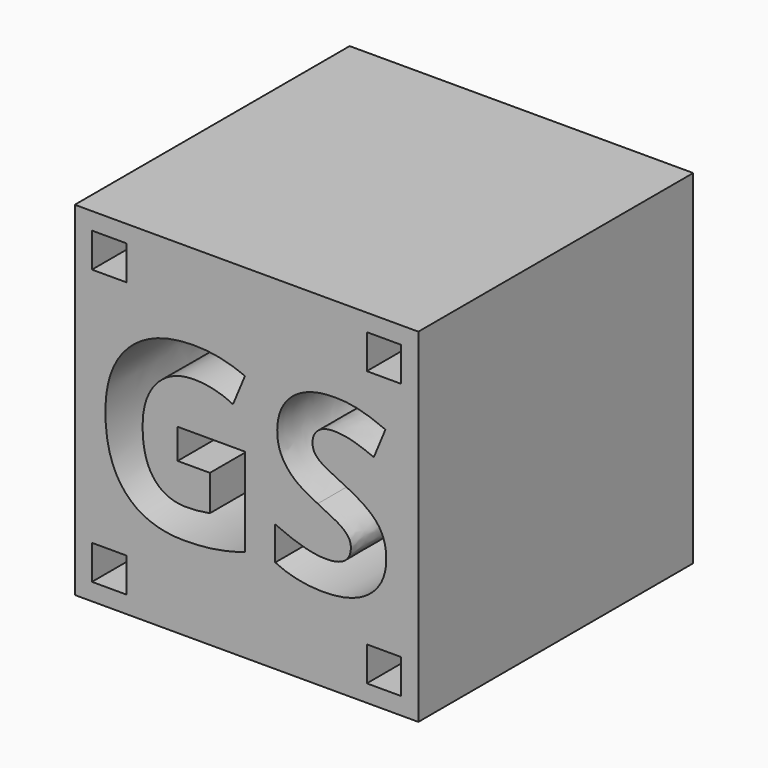
from build123d import *

# Parameters (mm, degrees)
F0_W         = 25.4
F0_H         = 25.4
F1_DEPTH     = 25.4
F2_TEXT_SIZE = 17.6388888889
F3_DEPTH     = 19.05
F4_W         = 2.54
F4_H         = 2.54
F5_DEPTH     = 6.35
F6_W         = 2.54
F6_H         = 2.54
F7_DEPTH     = 6.35
F8_W         = 2.54
F8_H         = 2.54
F9_DEPTH     = 6.35
F10_W        = 2.54
F10_H        = 2.54
F11_DEPTH    = 6.35
F12_W        = 22.86
F12_H        = 22.86
F13_DEPTH    = 6.35
F14_W        = 20.32
F14_H        = 3.81
F15_DEPTH    = 0.508


# Not quite as in the source:
# - Text() gives the source's letters only with a copy of the font that has no kerning and outlines rounded to 1/6400 em; it was checked with that copy


with BuildPart() as f1:
    # F0 (on Front) → F1 (new body)
    with BuildSketch(Plane.XZ):
        with Locations((1.8047373742, 0)):
            Rectangle(F0_W, F0_H)
    extrude(amount=F1_DEPTH)

    # F2 (on face) → F3 (cut)
    with BuildSketch(Plane.XZ.offset(25.4)):
        with Locations((-9.6569647978, -6.35)):
            Text('GS', F2_TEXT_SIZE, font='Open Sans', font_style=FontStyle.BOLD, text_align=(TextAlign.LEFT, TextAlign.BOTTOM))
    extrude(amount=-F3_DEPTH, mode=Mode.SUBTRACT)

    # F4 (on face) → F5 (cut)
    with BuildSketch(Plane.XZ.offset(25.4)):
        with Locations((-8.3552626258, 10.16)):
            Rectangle(F4_W, F4_H)
    extrude(amount=-F5_DEPTH, mode=Mode.SUBTRACT)

    # F6 (on face) → F7 (cut)
    with BuildSketch(Plane.XZ.offset(25.4)):
        with Locations((11.9647373742, 10.16)):
            Rectangle(F6_W, F6_H)
    extrude(amount=-F7_DEPTH, mode=Mode.SUBTRACT)

    # F8 (on face) → F9 (cut)
    with BuildSketch(Plane.XZ.offset(25.4)):
        with Locations((-8.3552626258, -10.16)):
            Rectangle(F8_W, F8_H)
    extrude(amount=-F9_DEPTH, mode=Mode.SUBTRACT)

    # F10 (on face) → F11 (cut)
    with BuildSketch(Plane.XZ.offset(25.4)):
        with Locations((11.9647373742, -10.16)):
            Rectangle(F10_W, F10_H)
    extrude(amount=-F11_DEPTH, mode=Mode.SUBTRACT)

    # F12 (on face) → F13 (cut)
    with BuildSketch(Plane(origin=(0, 0, 0), x_dir=(-1, 0, 0), z_dir=(0, 1, 0))):
        with Locations((-1.8047373742, 0)):
            Rectangle(F12_W, F12_H)
    extrude(amount=-F13_DEPTH, mode=Mode.SUBTRACT)

    # F14 (on face) → F15 (cut)
    with BuildSketch(Plane.XY.offset(-11.43)):
        with Locations((1.8047373742, -3.175)):
            Rectangle(F14_W, F14_H)
    extrude(amount=-F15_DEPTH, mode=Mode.SUBTRACT)


solid = f1.part
